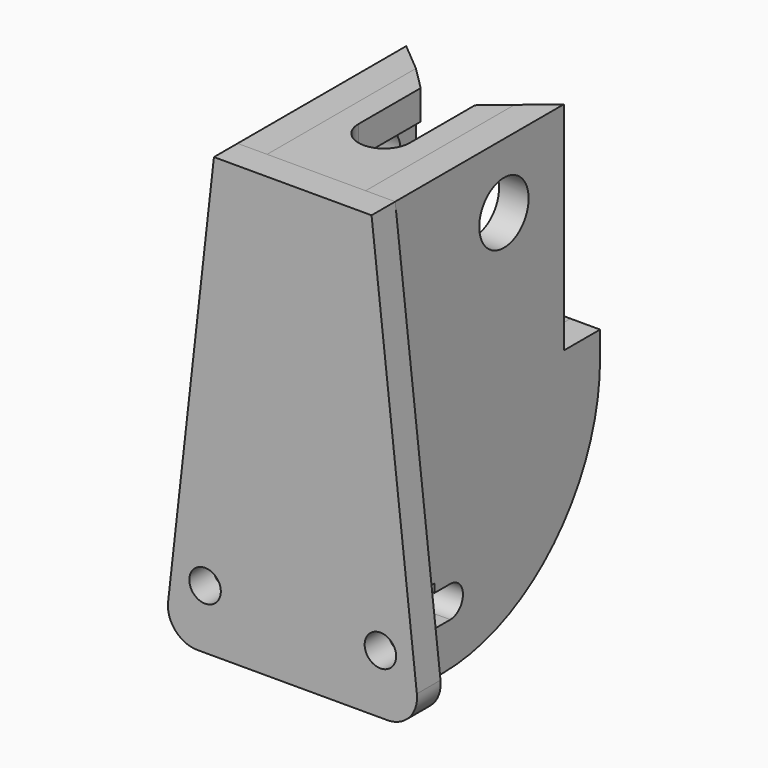
from build123d import *

# Parameters (mm, degrees)
F0_R      = 8
F1_DEPTH  = 15
F3_START  = 25
F2_R      = 15.6765625
F3_DEPTH  = 15
F4_SIZE2  = 12.586484
F4_SIZE   = 14.99999
F7_DEPTH  = 15
F8_SIZE2  = 10.069186
F8_SIZE   = 11.99999
F9_SIZE2  = 11.99999
F9_SIZE   = 11.99999
F11_START = -110
F11_DEPTH = 10


# Not quite as in the source:
# - a fillet or chamfer is up to 0.001 mm smaller than in the source, because OpenCascade refuses the exact size


with BuildPart() as f1:
    # F0 (on Front) → F1 (new body)
    with BuildSketch(Plane.XZ):
        with BuildLine():
            Line((-48.3547807248, -223), (0, -223))
            Line((0, -223), (48.0940515583, -223))
            ThreePointArc((48.0940515583, -223), (59.27277344, -218.001808691), (63.0017099144, -206.3381569454))
            Line((63.0017099144, -206.3381569454), (40, 0))
            Line((40, 0), (0, 0))
            Line((0, 0), (-40, 0))
            Line((-40, 0), (-63.2603535366, -206.3195538826))
            ThreePointArc((-63.2603535366, -206.3195538826), (-59.5397414257, -217.9948313702), (-48.3547807248, -223))
        make_face()
        with Locations((-44.5, -193)):
            Circle(F0_R, mode=Mode.SUBTRACT)
        with Locations((44.5, -193)):
            Circle(F0_R, mode=Mode.SUBTRACT)
    extrude(amount=F1_DEPTH)


with BuildPart() as f3:
    # F2 (on Right) → F3 (new body)
    with BuildSketch(Plane.YZ.offset(F3_START)):
        with BuildLine():
            Line((107, 0), (0, 0))
            Line((0, 0), (0, -180.75))
            Line((0, -180.75), (25, -180.75))
            Line((25, -180.75), (25, -185))
            Line((25, -185), (35, -185))
            ThreePointArc((35, -185), (43, -193), (35, -201))
            Line((35, -201), (25, -201))
            Line((25, -201), (25, -205.25))
            Line((25, -205.25), (0, -205.25))
            Line((0, -205.25), (0, -223))
            Line((0, -223), (30, -223))
            ThreePointArc((30, -223), (100.7106781187, -193.7106781187), (130, -123))
            Line((130, -123), (130, -110))
            Line((130, -110), (107, -110))
            Line((107, -110), (107, 0))
        make_face()
        with Locations((69, -33)):
            Circle(F2_R, mode=Mode.SUBTRACT)
    extrude(amount=F3_DEPTH)

    # F4 (size 15 and 12.5864944677 in the source; OpenCascade refuses exactly that, so slightly less here)
    f4_edges = [f3.edges().sort_by_distance(p)[0] for p in [
        (25, 107, -55),
    ]]
    f4_side = f3.faces().sort_by_distance((32.5, 107, -55))[0]
    chamfer(f4_edges, length=F4_SIZE, length2=F4_SIZE2, reference=f4_side)


with BuildPart() as f5_1:
    # F5: instance of F3
    add(f3.part.mirror(Plane.YZ))


with BuildPart() as f7:
    # F6 (on Top) → F7 (new body)
    with BuildSketch(Plane.XY):
        with BuildLine():
            Line((-25, 0), (0, 0))
            Line((0, 0), (25, 0))
            Line((25, 0), (25, 94.4135055323))
            Line((25, 94.4135055323), (13, 94.4135055323))
            Line((13, 94.4135055323), (13, 43))
            ThreePointArc((13, 43), (9.1923881554, 33.8076118446), (0, 30))
            ThreePointArc((0, 30), (-9.1923881554, 33.8076118446), (-13, 43))
            Line((-13, 43), (-13, 94.4135055323))
            Line((-13, 94.4135055323), (-25, 94.4135055323))
            Line((-25, 94.4135055323), (-25, 0))
        make_face()
    extrude(amount=-F7_DEPTH)

    # F8 (size 12 and 10.0691955741 in the source; OpenCascade refuses exactly that, so slightly less here)
    f8_edges = [f7.edges().sort_by_distance(p)[0] for p in [
        (13, 94.413506, -7.5),
    ]]
    f8_side = f7.faces().sort_by_distance((19, 94.413506, -7.5))[0]
    chamfer(f8_edges, length=F8_SIZE, length2=F8_SIZE2, reference=f8_side)

    # F9 (size 12 and 12 in the source; OpenCascade refuses exactly that, so slightly less here)
    f9_edges = [f7.edges().sort_by_distance(p)[0] for p in [
        (-13, 94.413506, -7.5),
    ]]
    chamfer(f9_edges, length=F9_SIZE, length2=F9_SIZE2)


with BuildPart() as f11:
    # F10 (on Top) → F11 (new body)
    with BuildSketch(Plane.XY.offset(F11_START)):
        Polygon((-25, 0), (0, 0), (25, 0), (25, 130), (-25, 130), align=None)
    extrude(amount=-F11_DEPTH)


solid = Compound([f1.part, f3.part, f5_1.part, f7.part, f11.part])
